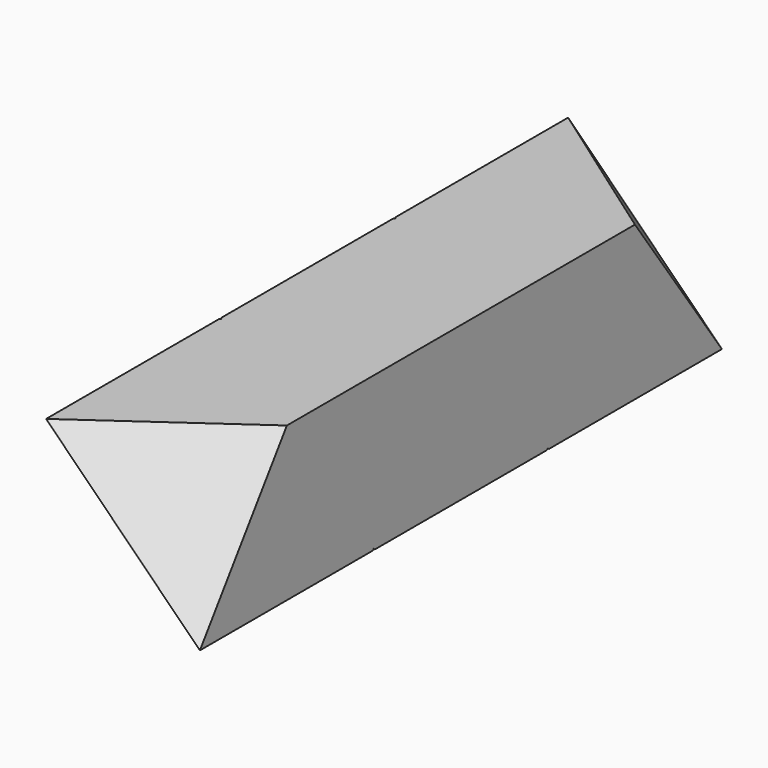
from build123d import *

# Parameters (mm, degrees)
F0_W     = 10.6066017178
F0_H     = 10.6066017178
F1_DEPTH = 22.5
F4_DEPTH = 15
F6_DEPTH = 15
F8_DEPTH = 15


# Not quite as in the source:
# - a feature names something its author has since deleted; it is built from what else it names


with BuildPart() as f1:
    # F0 (on Front) → F1 (new body, symmetric)
    with BuildSketch(Plane.XZ):
        Rectangle(F0_W, F0_H)
    extrude(amount=F1_DEPTH, both=True)

    # F3 (on 3pt) → F4 (cut, symmetric)
    with BuildSketch(Plane(origin=(0, 0, 0), x_dir=(0, 1, 0), z_dir=(0.7071067812, 0, -0.7071067812))):
        Polygon((-15, -7.5), (-22.5, 0), (-15, 7.5), (-15, 9.5), (-24.5, 9.5), (-24.5, -9.5), (-15, -9.5), align=None)
        Polygon((15, 7.5), (22.5, 0), (15, -7.5), (15, -9.5), (24.5, -9.5), (24.5, 9.5), (15, 9.5), align=None)
    extrude(amount=F4_DEPTH, both=True, mode=Mode.SUBTRACT)

    # F5 (on 3pt) → F6 (cut, symmetric)
    with BuildSketch(Plane(origin=(0, 0, 0), x_dir=(0, 1, 0), z_dir=(0.7071067812, 0, -0.7071067812))):
        Polygon((7.5, 0), (0, -7.5), (-7.5, 0), (-15, -7.5), (-15, -9.5), (15, -9.5), (15, -7.5), align=None)
    extrude(amount=F6_DEPTH, both=True, mode=Mode.SUBTRACT)

    # F7 (on 3pt) → F8 (cut, symmetric)
    with BuildSketch(Plane(origin=(0, 0, 0), x_dir=(0, 1, 0), z_dir=(0.7071067812, 0, -0.7071067812))):
        Polygon((-7.5, 0.0707106781), (-16.0707106781, -8.5), (16.0707106781, -8.5), (7.5, 0.0707106781), (0, -7.4292893219), align=None)
    extrude(amount=F8_DEPTH, both=True, mode=Mode.SUBTRACT)


solid = f1.part
